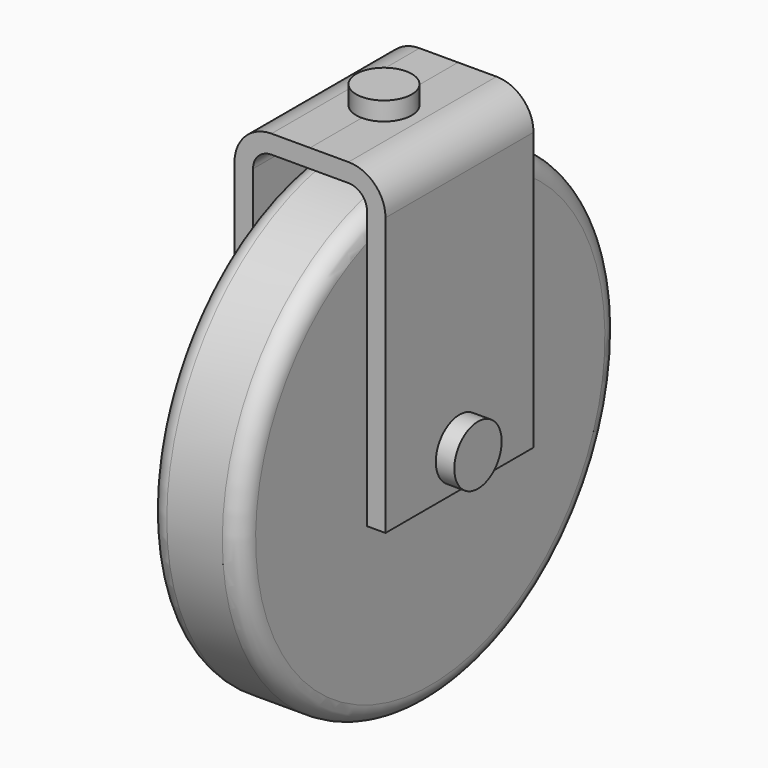
from build123d import *

# Parameters (mm, degrees)
F3_DEPTH = 25
F4_R     = 7.5
F5_DEPTH = 5


# Not quite as in the source:
# - ends of sketch curves that miss each other by under 0.0002 mm in the source are joined


with BuildPart() as f1:
    # F0 (on Front) → F1 (revolve)
    with BuildSketch(Plane.XZ):
        with BuildLine():
            Line((-20.4, 8), (-25.4, 8))
            Line((-25.4, 8), (-25.4, 0))
            Line((-25.4, 0), (-12.5, 0))
            Line((-12.5, 0), (12.5, 0))
            Line((12.5, 0), (25.4, 0))
            Line((25.4, 0), (25.4, 8))
            Line((25.4, 8), (20.4, 8))
            Line((20.4, 8), (20.4, 5))
            Line((20.4, 5), (15.4, 5))
            Line((15.4, 5), (15.4, 8))
            Line((15.4, 8), (12.5, 8))
            Line((12.5, 8), (12.5, 59))
            ThreePointArc((12.5, 59), (11.0355339059, 62.5355339059), (7.5, 64))
            Line((7.5, 64), (-7.5, 64))
            ThreePointArc((-7.5, 64), (-11.0355339059, 62.5355339059), (-12.5, 59))
            Line((-12.5, 59), (-12.5, 8))
            Line((-12.5, 8), (-15.4, 8))
            Line((-15.4, 8), (-15.4, 5))
            Line((-15.4, 5), (-20.4, 5))
            Line((-20.4, 5), (-20.4, 8))
        make_face()
    revolve(axis=Axis((-6.7645025283, 0, 0), (1, 0, 0)))

    # F2 (on Front) → F3 (join, symmetric)
    with BuildSketch(Plane.XZ):
        with BuildLine():
            Line((-20.4, -10), (-15.4, -10))
            Line((-15.4, -10), (-15.4, 65.000000298))
            ThreePointArc((-15.4, 65.000000298), (-13.9355339059, 68.535534204), (-10.4, 70.000000298))
            Line((-10.4, 70.000000298), (0, 70.000000298))
            Line((0, 70.000000298), (10.4, 70.000000298))
            ThreePointArc((10.4, 70.000000298), (13.9355339059, 68.535534204), (15.4, 65.000000298))
            Line((15.4, 65.000000298), (15.4, -10))
            Line((15.4, -10), (20.4, -10))
            Line((20.4, -10), (20.4, 65.000000298))
            ThreePointArc((20.4, 65.000000298), (17.4710678407, 72.0710681387), (10.4, 75.0000003388))
            Line((10.4, 75.0000003388), (0, 75))
            Line((0, 75), (-10.4, 75))
            ThreePointArc((-10.4, 75), (-17.4710678407, 72.0710681387), (-20.4000000408, 65.000000298))
            Line((-20.4000000408, 65.000000298), (-20.4, -10))
        make_face()
    extrude(amount=F3_DEPTH, both=True)

    # F4 (on face) → F5 (join)
    with BuildSketch(Plane.XY.offset(75)):
        Circle(F4_R)
    extrude(amount=F5_DEPTH)


solid = f1.part
